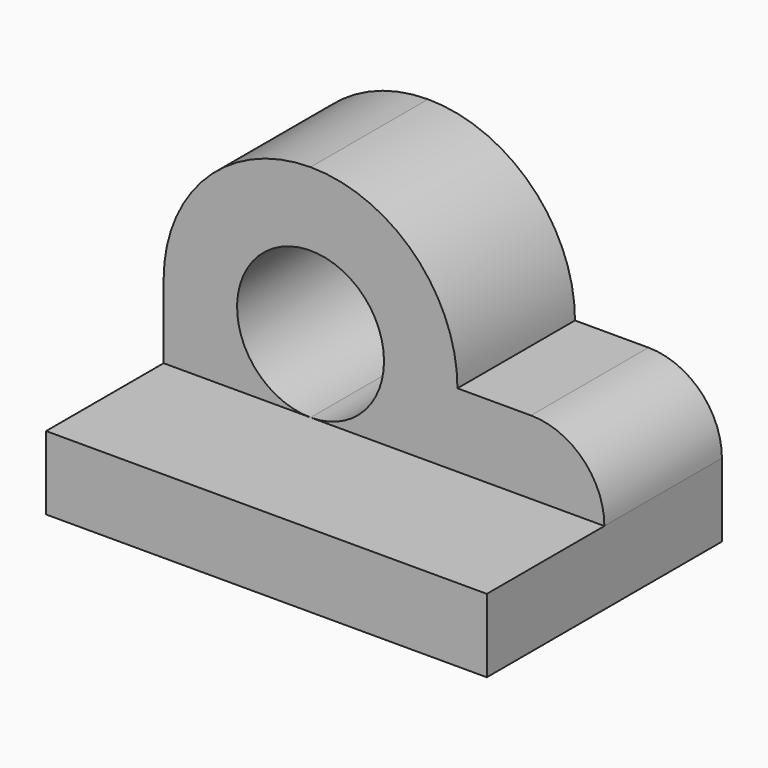
from build123d import *

# Parameters (mm, degrees)
F0_W     = 60
F0_H     = 40
F1_DEPTH = 10
F2_W     = 60
F2_H     = 20
F3_DEPTH = 10
F4_R     = 10
F5_W     = 40
F5_H     = 20
F6_DEPTH = 20
F8_DEPTH = 20
F9_R     = 19.99999


# Not quite as in the source:
# - a fillet or chamfer is up to 0.001 mm smaller than in the source, because OpenCascade refuses the exact size


with BuildPart() as f1:
    # F0 (on Top) → F1 (new body)
    with BuildSketch(Plane.XY):
        with Locations((2.6738010347, 9.0351510644)):
            Rectangle(F0_W, F0_H)
    extrude(amount=F1_DEPTH)

    # F2 (on face) → F3 (join)
    with BuildSketch(Plane.XY.offset(10)):
        with Locations((2.6738010347, 19.0351510644)):
            Rectangle(F2_W, F2_H)
    extrude(amount=F3_DEPTH)

    # F4
    f4_edges = [f1.edges().sort_by_distance(p)[0] for p in [
        (32.673801, 19.035151, 20),
    ]]
    fillet(f4_edges, radius=F4_R)

    # F5 (on face) → F6 (join)
    with BuildSketch(Plane.XY.offset(20)):
        with Locations((-7.3261989653, 19.0351510644)):
            Rectangle(F5_W, F5_H)
    extrude(amount=F6_DEPTH)

    # F7 (on face) → F8 (cut)
    with BuildSketch(Plane.XZ.offset(-9.0351510644)):
        with BuildLine():
            ThreePointArc((2.6738010347, 20), (-14.3972667772, 27.0710678119), (-7.3261989653, 10))
            ThreePointArc((-7.3261989653, 10), (-0.2551311534, 12.9289321881), (2.6738010347, 20))
        make_face()
    extrude(amount=-F8_DEPTH, mode=Mode.SUBTRACT)

    # F9 (radius 20 in the source; OpenCascade refuses exactly that, so slightly less here)
    f9_edges = [f1.edges().sort_by_distance(p)[0] for p in [
        (-27.326199, 19.035151, 40),
        (12.673801, 19.035151, 40),
    ]]
    fillet(f9_edges, radius=F9_R)


solid = f1.part
